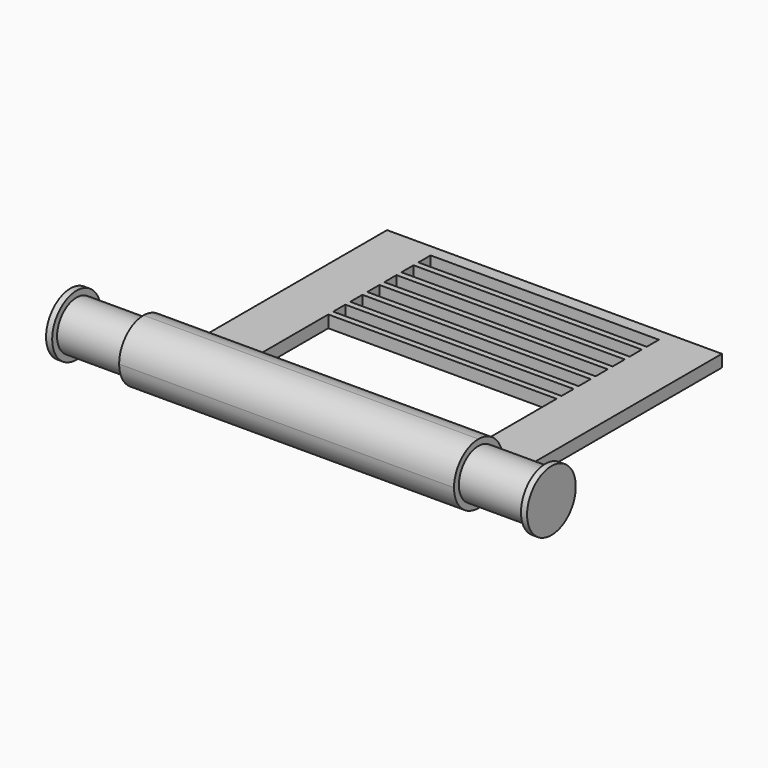
from build123d import *

# Parameters (mm, degrees)
F0_W     = 110
F0_H     = 20
F0_H_2   = 90
F1_DEPTH = 4
F2_DEPTH = 20
F4_DEPTH = 100
F3_R     = 8
F5_DEPTH = 77
F6_R     = 10
F6_R_2   = 8
F7_DEPTH = 2
F8_W     = 75
F8_H     = 5
F9_DEPTH = 25


# Not quite as in the source:
# - a pattern or mirror of a feature is missing from the dataset's text; its kind, count and spacing are read off the source's solid
# - a feature names something its author has since deleted; it is built from what else it names


with BuildPart() as f1:
    # F0 (on Top) → F1 (new body)
    with BuildSketch(Plane.XY):
        with Locations((0, -55)):
            Rectangle(F0_W, F0_H)
        Rectangle(F0_W, F0_H_2)
    extrude(amount=F1_DEPTH)

    # F0 (on Top) → F2 (join)
    with BuildSketch(Plane.XY):
        with Locations((0, -55)):
            Rectangle(F0_W, F0_H)
    extrude(amount=F2_DEPTH)

    # F3 (on Right) → F4 (cut, symmetric)
    with BuildSketch(Plane.YZ):
        with BuildLine():
            Line((-65, 2), (-65, 0))
            Line((-65, 0), (-55, 0))
            ThreePointArc((-55, 0), (-62.0710678119, 2.9289321881), (-65, 10))
            Line((-65, 10), (-65, 2))
        make_face()
        with BuildLine():
            Line((-65, 20), (-65, 10))
            ThreePointArc((-65, 10), (-62.0710678119, 17.0710678119), (-55, 20))
            Line((-55, 20), (-65, 20))
        make_face()
        with BuildLine():
            ThreePointArc((-55, 20), (-47.9289321881, 17.0710678119), (-45, 10))
            Line((-45, 10), (-45, 20))
            Line((-45, 20), (-55, 20))
        make_face()
    extrude(amount=F4_DEPTH, both=True, mode=Mode.SUBTRACT)

    # F3 (on Right) → F5 (join, symmetric)
    with BuildSketch(Plane.YZ):
        with Locations((-55, 10)):
            Circle(F3_R)
    extrude(amount=F5_DEPTH, both=True)

    # F6 (on face) → F7 (join)
    with BuildSketch(Plane(origin=(-77, 0, 0), x_dir=(0, -1, 0), z_dir=(-1, 0, 0))):
        with Locations((55, 10)):
            Circle(F6_R)
        with Locations((55, 10)):
            Circle(F6_R_2, mode=Mode.SUBTRACT)
        with Locations((55, 10)):
            Circle(F6_R_2)
    f7 = extrude(amount=F7_DEPTH)

    # F7_copies: F7 across plane
    add(f7.mirror(Plane(origin=(0, 0, 0), x_dir=(0, 0, 1), z_dir=(1, 0, 0))))

    # F8 (on face) → F9 (cut)
    with BuildSketch(Plane.XY.offset(4)):
        with Locations((0, 3.5)):
            Rectangle(F8_W, F8_H)
        with Locations((0, 10.5)):
            Rectangle(F8_W, F8_H)
        with Locations((0, 31.5)):
            Rectangle(F8_W, F8_H)
        with Locations((0, 24.5)):
            Rectangle(F8_W, F8_H)
        with Locations((0, 17.5)):
            Rectangle(F8_W, F8_H)
        with Locations((0, 38.5)):
            Rectangle(F8_W, F8_H)
        Polygon((37.5, -8), (37.5, -6), (37.5, -1), (-37.5, -1), (-37.5, -6), (-37.5, -8), (-37.5, -13), (-37.5, -15), (-37.5, -20), (-37.5, -22), (-37.5, -27), (-37.5, -29), (-37.5, -34), (-37.5, -36), (-37.5, -41), (37.5, -41), (37.5, -36), (37.5, -34), (37.5, -29), (37.5, -27), (37.5, -22), (37.5, -20), (37.5, -15), (37.5, -13), align=None)
    extrude(amount=-F9_DEPTH, mode=Mode.SUBTRACT)


solid = f1.part
